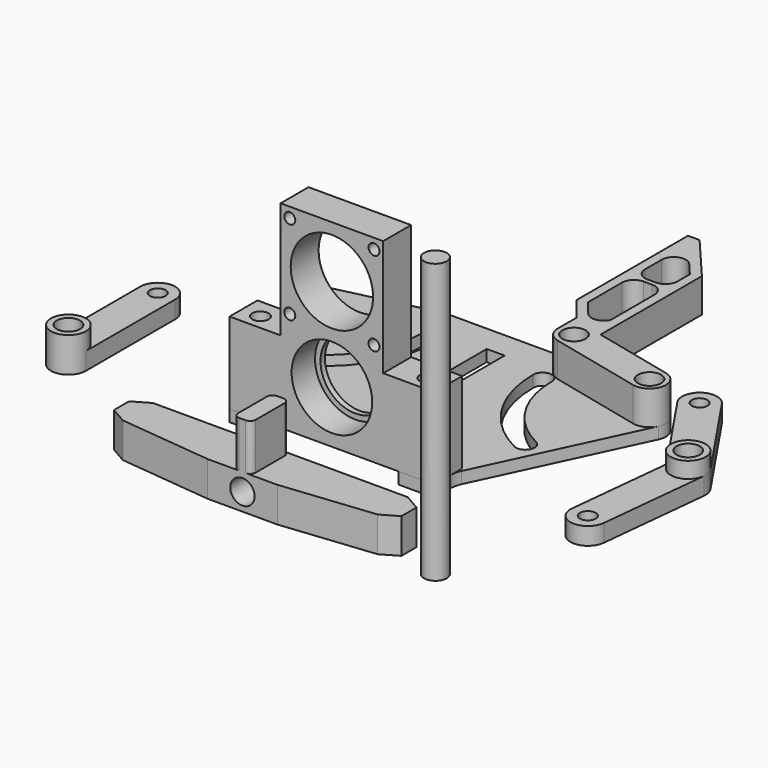
from build123d import *

# Parameters (mm, degrees)
F0_R      = 2.5527
F0_R_2    = 2.2479
F1_DEPTH  = 3.175
F2_R      = 2.159
F2_R_2    = 3.175
F3_DEPTH  = 4.7625
F4_R      = 2.159
F4_R_2    = 3.175
F5_DEPTH  = 4.7625
F6_R      = 3.175
F7_DEPTH  = 9.271
F8_W      = 55.88
F8_H      = 9.525
F8_R      = 2.2479
F9_DEPTH  = 22.225
F10_W     = 28
F10_H     = 9.525
F11_DEPTH = 31.75
F12_R     = 11
F13_DEPTH = 8
F14_R     = 9.525
F15_DEPTH = 101.602
F16_R     = 11.25
F16_R_2   = 1.5
F17_DEPTH = 14.9194730585
F19_DEPTH = 9.525
F20_R     = 3.31978
F21_DEPTH = 140.1346438931
F22_R     = 3.10261
F23_DEPTH = 76.2
F25_DEPTH = 0.0254
F27_DEPTH = 12.7
F28_R     = 4.7625
F28_R_2   = 3.175
F29_DEPTH = 4.7625
F30_R     = 4.7633639438
F30_R_2   = 3.175
F31_DEPTH = 4.3815
F33_DEPTH = 12.447


# Not quite as in the source:
# - ends of sketch curves that miss each other by under 0.0002 mm in the source are joined


with BuildPart() as f1:
    # F0 (on Top) → F1 (new body)
    with BuildSketch(Plane.XY):
        with BuildLine():
            Line((19.05, 63.246), (-19.05, 63.246))
            ThreePointArc((-19.05, 63.246), (-19.5618416502, 63.2164323826), (-20.0668738794, 63.128122891))
            Line((-20.0668738794, 63.128122891), (-45.4668738794, 57.159122891))
            ThreePointArc((-45.4668738794, 57.159122891), (-48.451322506, 54.7678313983), (-48.4739277117, 50.9436062986))
            Line((-48.4739277117, 50.9436062986), (-28.5655931141, 8.5214677257))
            ThreePointArc((-28.5655931141, 8.5214677257), (-28.0982954196, 7.1531114974), (-27.94, 5.7158542265))
            Line((-27.94, 5.7158542265), (-27.94, 0))
            Line((-27.94, 0), (-18.161, 0))
            Line((-18.161, 0), (-18.161, 9.525))
            Line((-18.161, 9.525), (-2.44475, 9.525))
            Line((-2.44475, 9.525), (-2.44475, 55.889925157))
            Line((-2.44475, 55.889925157), (2.44475, 55.889925157))
            Line((2.44475, 55.889925157), (2.44475, 9.525))
            Line((2.44475, 9.525), (18.161, 9.525))
            Line((18.161, 9.525), (18.161, 0))
            Line((18.161, 0), (27.94, 0))
            Line((27.94, 0), (27.94, 5.7158542265))
            ThreePointArc((27.94, 5.7158542265), (28.0982954196, 7.1531114974), (28.5655931141, 8.5214677257))
            Line((28.5655931141, 8.5214677257), (48.4739277117, 50.9436062986))
            ThreePointArc((48.4739277117, 50.9436062986), (48.451322506, 54.7678313983), (45.4668738794, 57.159122891))
            Line((45.4668738794, 57.159122891), (20.0668738794, 63.128122891))
            ThreePointArc((20.0668738794, 63.128122891), (19.5618416502, 63.2164323826), (19.05, 63.246))
        make_face()
        with Locations((-22.86, 4.191)):
            Circle(F0_R, mode=Mode.SUBTRACT)
        with Locations((22.86, 4.191)):
            Circle(F0_R, mode=Mode.SUBTRACT)
        with BuildLine():
            ThreePointArc((-12.7, 52.832), (-17.4679645864, 36.0978353977), (-30.3398277126, 24.3896805091))
            ThreePointArc((-30.3398277126, 24.3896805091), (-33.7440270549, 25.5362522854), (-32.5974552786, 28.9404516277))
            ThreePointArc((-32.5974552786, 28.9404516277), (-21.7850902526, 38.775301734), (-17.78, 52.832))
            ThreePointArc((-17.78, 52.832), (-15.24, 55.372), (-12.7, 52.832))
        make_face(mode=Mode.SUBTRACT)
        with Locations((-44.45, 52.832)):
            Circle(F0_R_2, mode=Mode.SUBTRACT)
        with Locations((-19.05, 58.801)):
            Circle(F0_R_2, mode=Mode.SUBTRACT)
        with BuildLine():
            ThreePointArc((12.7, 52.832), (15.24, 55.372), (17.78, 52.832))
            ThreePointArc((17.78, 52.832), (21.7850902526, 38.775301734), (32.5974552786, 28.9404516277))
            ThreePointArc((32.5974552786, 28.9404516277), (33.7440270549, 25.5362522854), (30.3398277126, 24.3896805091))
            ThreePointArc((30.3398277126, 24.3896805091), (17.4679645864, 36.0978353977), (12.7, 52.832))
        make_face(mode=Mode.SUBTRACT)
        with Locations((19.05, 58.801)):
            Circle(F0_R_2, mode=Mode.SUBTRACT)
        with Locations((44.45, 52.832)):
            Circle(F0_R_2, mode=Mode.SUBTRACT)
    extrude(amount=F1_DEPTH)


with BuildPart() as f3:
    # F2 (on Top) → F3 (new body)
    with BuildSketch(Plane.XY):
        with BuildLine():
            ThreePointArc((-76.1907740574, 29.8490269415), (-71.4282740574, 25.0865269415), (-66.6657740574, 29.8490269415))
            ThreePointArc((-66.6657740574, 29.8490269415), (-71.4282740574, 34.6115269415), (-76.1907740574, 29.8490269415))
        make_face()
        with Locations((-71.4282740574, 29.8490269415)):
            Circle(F2_R, mode=Mode.SUBTRACT)
        with BuildLine():
            Line((-66.6657740574, -0.6309730585), (-66.6657740574, 29.8490269415))
            ThreePointArc((-66.6657740574, 29.8490269415), (-71.4282740574, 25.0865269415), (-76.1907740574, 29.8490269415))
            Line((-76.1907740574, 29.8490269415), (-76.1907740574, -0.6309730585))
            ThreePointArc((-76.1907740574, -0.6309730585), (-71.4282740574, 4.1315269415), (-66.6657740574, -0.6309730585))
        make_face()
        with BuildLine():
            ThreePointArc((-76.1907740574, -0.6309730585), (-71.4282740574, -5.3934730585), (-66.6657740574, -0.6309730585))
            ThreePointArc((-66.6657740574, -0.6309730585), (-71.4282740574, 4.1315269415), (-76.1907740574, -0.6309730585))
        make_face()
        with Locations((-71.4282740574, -0.6309730585)):
            Circle(F2_R_2, mode=Mode.SUBTRACT)
    extrude(amount=F3_DEPTH)

    # F28 (on face) → F29 (join)
    with BuildSketch(Plane.XY.offset(4.7625)):
        with Locations((-71.4282740574, -0.6309730585)):
            Circle(F28_R)
        with Locations((-71.4282740574, -0.6309730585)):
            Circle(F28_R_2, mode=Mode.SUBTRACT)
    extrude(amount=F29_DEPTH)


with BuildPart() as f5:
    # F4 (on Top) → F5 (new body)
    with BuildSketch(Plane.XY):
        with BuildLine():
            Line((71.4840174561, 39.834444246), (54.402320682, 65.0781768409))
            ThreePointArc((54.402320682, 65.0781768409), (47.7877726452, 66.3537262876), (46.5122231985, 59.7391782508))
            Line((46.5122231985, 59.7391782508), (62.6223016887, 35.9313259707))
            Line((62.6223016887, 35.9313259707), (59.6599453355, 7.3380941843))
            ThreePointArc((59.6599453355, 7.3380941843), (64.6437130785, 11.6042405017), (69.1613130167, 6.8472208344))
            ThreePointArc((69.1613130167, 6.8472208344), (69.1551738197, 6.6054590305), (69.1367720534, 6.3643204094))
            Line((69.1367720534, 6.3643204094), (72.2769724517, 36.674071601))
            ThreePointArc((72.2769724517, 36.674071601), (72.1591244371, 38.3241676037), (71.4840174561, 39.834444246))
        make_face()
        with Locations((50.4572719402, 62.4086775458)):
            Circle(F4_R, mode=Mode.SUBTRACT)
        with Locations((67.5389687143, 37.164944951)):
            Circle(F4_R_2, mode=Mode.SUBTRACT)
        with BuildLine():
            ThreePointArc((69.1613130167, 6.8472208344), (64.6437130785, 11.6042405017), (59.6599453355, 7.3380941843))
            ThreePointArc((59.6599453355, 7.3380941843), (63.9110620131, 2.1088057985), (69.1367720534, 6.3643204094))
            ThreePointArc((69.1367720534, 6.3643204094), (69.1551738197, 6.6054590305), (69.1613130167, 6.8472208344))
        make_face()
        with Locations((64.3979490729, 6.8472208344)):
            Circle(F4_R, mode=Mode.SUBTRACT)
    extrude(amount=F5_DEPTH)

    # F30 (on face) → F31 (join)
    with BuildSketch(Plane.XY.offset(4.7625)):
        with Locations((67.5389687143, 37.164944951)):
            Circle(F30_R)
        with Locations((67.5389687143, 37.164944951)):
            Circle(F30_R_2, mode=Mode.SUBTRACT)
    extrude(amount=F31_DEPTH)


with BuildPart() as f7:
    # F6 (on face) → F7 (new body)
    with BuildSketch(Plane.XY.offset(3.175)):
        with BuildLine():
            Line((18.0331261206, 54.473877109), (43.4331261206, 48.504877109))
            ThreePointArc((43.4331261206, 48.504877109), (48.777122891, 51.8151261206), (45.4668738794, 57.159122891))
            Line((45.4668738794, 57.159122891), (23.495, 62.3225132526))
            Line((23.495, 62.3225132526), (23.495, 58.801))
            ThreePointArc((23.495, 58.801), (21.8102554779, 55.3168911187), (18.0331261206, 54.473877109))
        make_face()
        with Locations((44.45, 52.832)):
            Circle(F6_R, mode=Mode.SUBTRACT)
        with BuildLine():
            ThreePointArc((14.605, 58.801), (15.5658911187, 56.0407445221), (18.0331261206, 54.473877109))
            ThreePointArc((18.0331261206, 54.473877109), (21.8102554779, 55.3168911187), (23.495, 58.801))
            Line((23.495, 58.801), (23.495, 62.3225132526))
            Line((23.495, 62.3225132526), (23.495, 96.901))
            Line((23.495, 96.901), (12.7, 109.601))
            Line((12.7, 109.601), (9.525, 109.601))
            Line((9.525, 109.601), (9.525, 71.501))
            Line((9.525, 71.501), (14.605, 65.151))
            Line((14.605, 65.151), (14.605, 58.801))
        make_face()
        with Locations((19.05, 58.801)):
            Circle(F6_R, mode=Mode.SUBTRACT)
    extrude(amount=F7_DEPTH)

    # F32 (on face) → F33 (cut, through all)
    with BuildSketch(Plane.XY.offset(12.446)):
        with BuildLine():
            Line((12.065, 83.8946654219), (12.065, 72.3919838908))
            Line((12.065, 72.3919838908), (15.353200649, 68.2817330795))
            ThreePointArc((15.353200649, 68.2817330795), (18.3612969836, 67.0705503764), (20.955, 69.0169089665))
            Line((20.955, 69.0169089665), (20.955, 83.8946654219))
            ThreePointArc((20.955, 83.8946654219), (19.9878665915, 86.2295320133), (17.653, 87.1966654219))
            Line((17.653, 87.1966654219), (15.367, 87.1966654219))
            ThreePointArc((15.367, 87.1966654219), (13.0321334085, 86.2295320133), (12.065, 83.8946654219))
        make_face()
        with BuildLine():
            Line((20.955, 91.7686654219), (20.955, 95.9673543458))
            Line((20.955, 95.9673543458), (17.8829236272, 99.5815618431))
            ThreePointArc((17.8829236272, 99.5815618431), (14.2277844403, 100.5422834303), (12.065, 97.44302676))
            Line((12.065, 97.44302676), (12.065, 91.7686654219))
            ThreePointArc((12.065, 91.7686654219), (13.0321334085, 89.4337988304), (15.367, 88.4666654219))
            Line((15.367, 88.4666654219), (17.653, 88.4666654219))
            ThreePointArc((17.653, 88.4666654219), (19.9878665915, 89.4337988304), (20.955, 91.7686654219))
        make_face()
    extrude(amount=-F33_DEPTH, mode=Mode.SUBTRACT)


with BuildPart() as f9:
    # F8 (on face) → F9 (new body)
    with BuildSketch(Plane.XY.offset(3.175)):
        with Locations((0, 4.7625)):
            Rectangle(F8_W, F8_H)
        with Locations((-22.86, 4.191)):
            Circle(F8_R, mode=Mode.SUBTRACT)
        with Locations((22.86, 4.191)):
            Circle(F8_R, mode=Mode.SUBTRACT)
    extrude(amount=F9_DEPTH)

    # F10 (on face) → F11 (join)
    with BuildSketch(Plane.XY.offset(25.4)):
        with Locations((0, 4.7625)):
            Rectangle(F10_W, F10_H)
    extrude(amount=F11_DEPTH)

    # F12 (on face) → F13 (cut)
    with BuildSketch(Plane.XZ):
        with Locations((0, 17.4625)):
            Circle(F12_R)
    extrude(amount=-F13_DEPTH, mode=Mode.SUBTRACT)

    # F14 (on face) → F15 (cut, through all)
    with BuildSketch(Plane.XZ.offset(-8)):
        with Locations((0, 17.4625)):
            Circle(F14_R)
    extrude(amount=-F15_DEPTH, mode=Mode.SUBTRACT)

    # F16 (on face) → F17 (cut, through all)
    with BuildSketch(Plane(origin=(0, 9.525, 0), x_dir=(-1, 0, 0), z_dir=(0, 1, 0))):
        with Locations((0, 42.8625)):
            Circle(F16_R)
        with Locations((11.5, 54.3625)):
            Circle(F16_R_2)
        with Locations((11.5, 31.3625)):
            Circle(F16_R_2)
        with Locations((-11.5, 31.3625)):
            Circle(F16_R_2)
        with Locations((-11.5, 54.3625)):
            Circle(F16_R_2)
    extrude(amount=-F17_DEPTH, mode=Mode.SUBTRACT)


with BuildPart() as f19:
    # F18 (on Top) → F19 (new body)
    with BuildSketch(Plane.XY):
        Polygon((-39.2308561424, -25.3112989795), (-34.7858561424, -27.8776209261), (-9.525, -30.5326438931), (9.525, -30.5326438931), (34.7858561424, -27.8776209261), (39.2308561424, -25.3112989795), (39.2308561424, -20.1786550865), (34.7858561424, -17.6123331399), (-34.7858561424, -17.6123331399), (-39.2308561424, -20.1786550865), align=None)
        with BuildLine():
            ThreePointArc((-9.1798470143, -22.1160887015), (-6.2410887015, -25.7451529857), (-9.8701529857, -28.6839112985))
            Line((-9.8701529857, -28.6839112985), (-35.1310091281, -26.0288883315))
            ThreePointArc((-35.1310091281, -26.0288883315), (-38.0697674409, -22.3998240473), (-34.4407031566, -19.4610657345))
            Line((-34.4407031566, -19.4610657345), (-9.1798470143, -22.1160887015))
        make_face(mode=Mode.SUBTRACT)
        with BuildLine():
            ThreePointArc((9.8701529857, -28.6839112985), (6.2410887015, -25.7451529857), (9.1798470143, -22.1160887015))
            Line((9.1798470143, -22.1160887015), (34.4407031566, -19.4610657345))
            ThreePointArc((34.4407031566, -19.4610657345), (38.0697674409, -22.3998240473), (35.1310091281, -26.0288883315))
            Line((35.1310091281, -26.0288883315), (9.8701529857, -28.6839112985))
        make_face(mode=Mode.SUBTRACT)
    extrude(amount=F19_DEPTH)

    # F20 (on face) → F21 (cut, through all)
    with BuildSketch(Plane.XZ.offset(30.5326438931)):
        with Locations((0, 4.7625)):
            Circle(F20_R)
    extrude(amount=-F21_DEPTH, mode=Mode.SUBTRACT)

    # F24 (on face) → F25 (join)
    with BuildSketch(Plane.XY.offset(9.525)):
        Polygon((-34.7858561424, -27.8776209261), (-9.525, -30.5326438931), (9.525, -30.5326438931), (34.7858561424, -27.8776209261), (39.2308561424, -25.3112989795), (39.2308561424, -20.1786550865), (34.7858561424, -17.6123331399), (-34.7858561424, -17.6123331399), (-39.2308561424, -20.1786550865), (-39.2308561424, -25.3112989795), align=None)
    extrude(amount=F25_DEPTH)

    # F26 (on face) → F27 (join)
    with BuildSketch(Plane.XY.offset(9.5504)):
        with BuildLine():
            Line((-0.889, -30.5326438931), (0.889, -30.5326438931))
            ThreePointArc((0.889, -30.5326438931), (1.9666307345, -30.0862746276), (2.413, -29.0086438931))
            Line((2.413, -29.0086438931), (2.413, -19.1363331399))
            ThreePointArc((2.413, -19.1363331399), (1.9666307345, -18.0587024054), (0.889, -17.6123331399))
            Line((0.889, -17.6123331399), (-0.889, -17.6123331399))
            ThreePointArc((-0.889, -17.6123331399), (-1.9666307345, -18.0587024054), (-2.413, -19.1363331399))
            Line((-2.413, -19.1363331399), (-2.413, -29.0086438931))
            ThreePointArc((-2.413, -29.0086438931), (-1.9666307345, -30.0862746276), (-0.889, -30.5326438931))
        make_face()
    extrude(amount=F27_DEPTH)


with BuildPart() as f23:
    # F22 (on Top) → F23 (new body)
    with BuildSketch(Plane.XY):
        with Locations((50.1387342811, -27.3660663515)):
            Circle(F22_R)
    extrude(amount=F23_DEPTH)


solid = Compound([f1.part, f3.part, f5.part, f7.part, f9.part, f19.part, f23.part])
